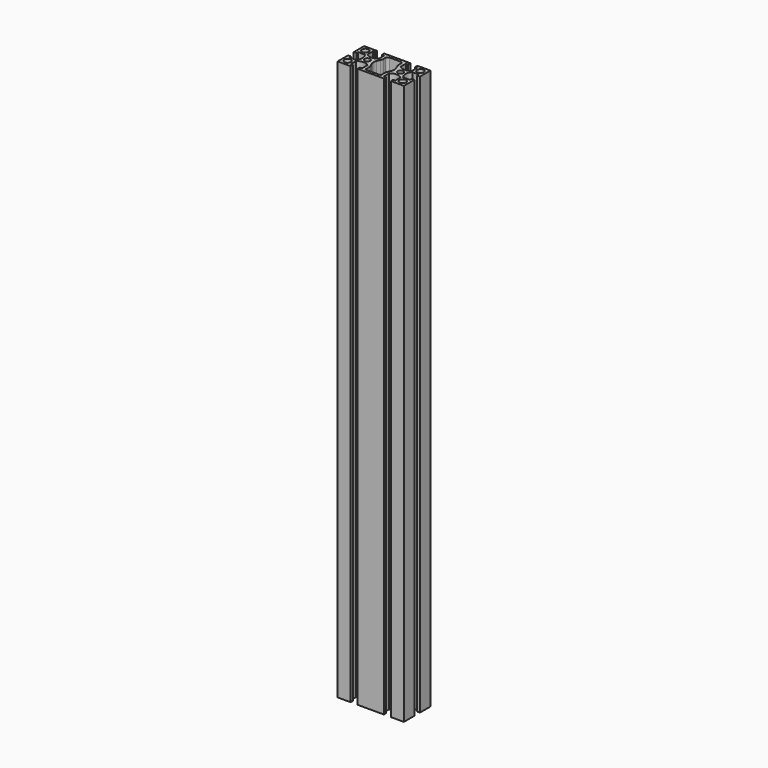
from build123d import *

# Parameters (mm, degrees)
F0_R     = 3
F0_R_2   = 2.5
F1_DEPTH = 507
F2_R     = 2
F3_R     = 7


# Not quite as in the source:
# - a feature names something its author has since deleted; it is built from what else it names


with BuildPart() as f1:
    # F0 (on Top) → F1 (new body)
    with BuildSketch(Plane.XY):
        with BuildLine():
            Line((18.15, -15), (30, -15))
            Line((30, -15), (30, -3.15))
            Line((30, -3.15), (27.5, -3.15))
            Line((27.5, -3.15), (27.5, -5.15))
            Line((27.5, -5.15), (21.5477069044, -5.15))
            ThreePointArc((21.5477069044, -5.15), (19.5, 0), (21.5477069044, 5.15))
            Line((21.5477069044, 5.15), (27.5, 5.15))
            Line((27.5, 5.15), (27.5, 3.15))
            Line((27.5, 3.15), (30, 3.15))
            Line((30, 3.15), (30, 15))
            Line((30, 15), (18.15, 15))
            Line((18.15, 15), (18.15, 12.5))
            Line((18.15, 12.5), (20.15, 12.5))
            Line((20.15, 12.5), (20.15, 6.5477069044))
            ThreePointArc((20.15, 6.5477069044), (15, 4.5), (9.85, 6.5477069044))
            Line((9.85, 6.5477069044), (9.85, 12.5))
            Line((9.85, 12.5), (11.85, 12.5))
            Line((11.85, 12.5), (11.85, 15))
            Line((11.85, 15), (-11.85, 15))
            Line((-11.85, 15), (-11.85, 12.5))
            Line((-11.85, 12.5), (-9.85, 12.5))
            Line((-9.85, 12.5), (-9.85, 6.5477069044))
            ThreePointArc((-9.85, 6.5477069044), (-15, 4.5), (-20.15, 6.5477069044))
            Line((-20.15, 6.5477069044), (-20.15, 12.5))
            Line((-20.15, 12.5), (-18.15, 12.5))
            Line((-18.15, 12.5), (-18.15, 15))
            Line((-18.15, 15), (-30, 15))
            Line((-30, 15), (-30, 3.15))
            Line((-30, 3.15), (-27.5, 3.15))
            Line((-27.5, 3.15), (-27.5, 5.15))
            Line((-27.5, 5.15), (-21.5477069044, 5.15))
            ThreePointArc((-21.5477069044, 5.15), (-19.5, 0), (-21.5477069044, -5.15))
            Line((-21.5477069044, -5.15), (-27.5, -5.15))
            Line((-27.5, -5.15), (-27.5, -3.15))
            Line((-27.5, -3.15), (-30, -3.15))
            Line((-30, -3.15), (-30, -15))
            Line((-30, -15), (-18.15, -15))
            Line((-18.15, -15), (-18.15, -12.5))
            Line((-18.15, -12.5), (-20.15, -12.5))
            Line((-20.15, -12.5), (-20.15, -6.5477069044))
            ThreePointArc((-20.15, -6.5477069044), (-15, -4.5), (-9.85, -6.5477069044))
            Line((-9.85, -6.5477069044), (-9.85, -12.5))
            Line((-9.85, -12.5), (-11.85, -12.5))
            Line((-11.85, -12.5), (-11.85, -15))
            Line((-11.85, -15), (11.85, -15))
            Line((11.85, -15), (11.85, -12.5))
            Line((11.85, -12.5), (9.85, -12.5))
            Line((9.85, -12.5), (9.85, -6.5477069044))
            ThreePointArc((9.85, -6.5477069044), (15, -4.5), (20.15, -6.5477069044))
            Line((20.15, -6.5477069044), (20.15, -12.5))
            Line((20.15, -12.5), (18.15, -12.5))
            Line((18.15, -12.5), (18.15, -15))
        make_face()
        with Locations((-25, -10)):
            Circle(F0_R, mode=Mode.SUBTRACT)
        with Locations((25, -10)):
            Circle(F0_R, mode=Mode.SUBTRACT)
        with Locations((-15, 0)):
            Circle(F0_R_2, mode=Mode.SUBTRACT)
        with Locations((-25, 10)):
            Circle(F0_R, mode=Mode.SUBTRACT)
        Polygon((-7, 7), (-7, 12.5), (0, 12.5), (7, 12.5), (7, 7), (10, 0), (7, -7), (7, -12.5), (0, -12.5), (-7, -12.5), (-7, -7), (-10, 0), align=None, mode=Mode.SUBTRACT)
        with Locations((15, 0)):
            Circle(F0_R_2, mode=Mode.SUBTRACT)
        with Locations((25, 10)):
            Circle(F0_R, mode=Mode.SUBTRACT)
    extrude(amount=F1_DEPTH)

    # F2
    f2_edges = [f1.edges().sort_by_distance(p)[0] for p in [
        (-7, 12.5, 253.5),
        (7, 12.5, 253.5),
    ]]
    fillet(f2_edges, radius=F2_R)

    # F3
    f3_edges = [f1.edges().sort_by_distance(p)[0] for p in [
        (-7, 7, 253.5),
        (-10, 0, 253.5),
        (7, 7, 253.5),
        (10, 0, 253.5),
    ]]
    fillet(f3_edges, radius=F3_R)


solid = f1.part
